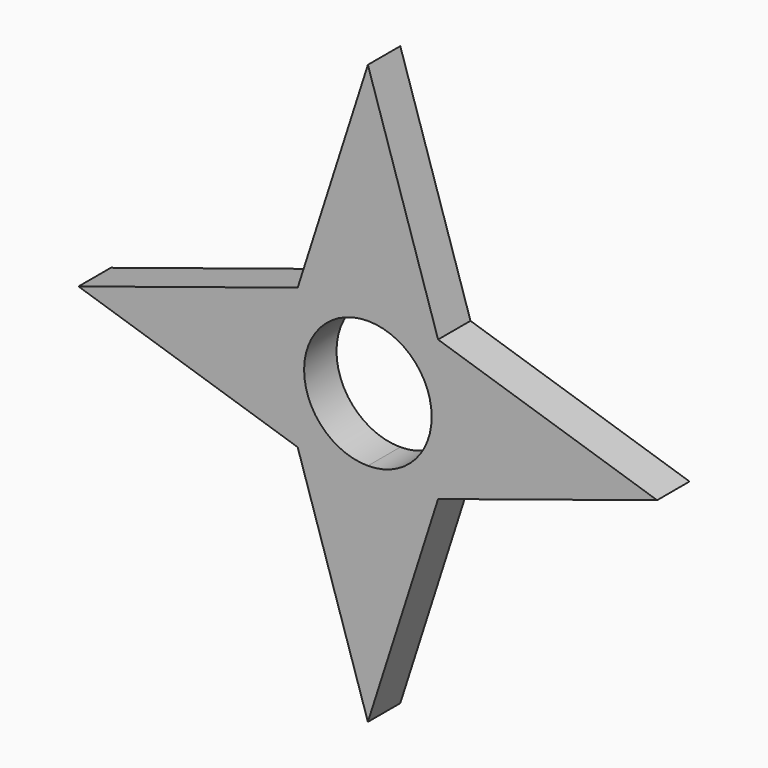
from build123d import *

# Parameters (mm, degrees)
F1_DEPTH = 7


with BuildPart() as f1:
    # F0 (on Front) → F1 (new body)
    with BuildSketch(Plane.XZ):
        with BuildLine():
            Line((13.0394884775, 9.315168557), (16.025, 0))
            ThreePointArc((16.025, 0), (15.2603805302, 4.8909519599), (13.0394884775, 9.315168557))
        make_face()
        with BuildLine():
            ThreePointArc((13.0394884775, 9.315168557), (15.2603805302, 4.8909519599), (16.025, 0))
            ThreePointArc((16.025, 0), (15.2603805302, -4.8909519599), (13.0394884775, -9.315168557))
            Line((13.0394884775, -9.315168557), (12.1355547141, -12.1355547141))
            Line((12.1355547141, -12.1355547141), (50, 0))
            Line((50, 0), (12.1355547141, 12.1355547141))
            Line((12.1355547141, 12.1355547141), (13.0394884775, 9.315168557))
        make_face()
        with BuildLine():
            Line((11.025, 0), (16.025, 0))
            Line((16.025, 0), (13.0394884775, 9.315168557))
            ThreePointArc((13.0394884775, 9.315168557), (11.3313861685, 11.3313861685), (9.315168557, 13.0394884775))
            Line((9.315168557, 13.0394884775), (0, 16.025))
            Line((0, 16.025), (0, 11.025))
            ThreePointArc((0, 11.025), (7.7958522626, 7.7958522626), (11.025, 0))
        make_face()
        with BuildLine():
            ThreePointArc((13.0394884775, -9.315168557), (15.2603805302, -4.8909519599), (16.025, 0))
            Line((16.025, 0), (13.0394884775, -9.315168557))
        make_face()
        with BuildLine():
            Line((13.0394884775, -9.315168557), (16.025, 0))
            Line((16.025, 0), (11.025, 0))
            ThreePointArc((11.025, 0), (7.7958522626, -7.7958522626), (0, -11.025))
            Line((0, -11.025), (0, -16.025))
            Line((0, -16.025), (9.315168557, -13.0394884775))
            ThreePointArc((9.315168557, -13.0394884775), (11.3313861685, -11.3313861685), (13.0394884775, -9.315168557))
        make_face()
        with BuildLine():
            ThreePointArc((9.315168557, 13.0394884775), (11.3313861685, 11.3313861685), (13.0394884775, 9.315168557))
            Line((13.0394884775, 9.315168557), (12.1355547141, 12.1355547141))
            Line((12.1355547141, 12.1355547141), (9.315168557, 13.0394884775))
        make_face()
        with BuildLine():
            Line((12.1355547141, -12.1355547141), (13.0394884775, -9.315168557))
            ThreePointArc((13.0394884775, -9.315168557), (11.3313861685, -11.3313861685), (9.315168557, -13.0394884775))
            Line((9.315168557, -13.0394884775), (12.1355547141, -12.1355547141))
        make_face()
        with BuildLine():
            Line((0, 16.025), (9.315168557, 13.0394884775))
            ThreePointArc((9.315168557, 13.0394884775), (4.8909519599, 15.2603805302), (0, 16.025))
        make_face()
        with BuildLine():
            ThreePointArc((0, 16.025), (4.8909519599, 15.2603805302), (9.315168557, 13.0394884775))
            Line((9.315168557, 13.0394884775), (12.1355547141, 12.1355547141))
            Line((12.1355547141, 12.1355547141), (0, 50))
            Line((0, 50), (-12.1347763783, 12.1379832191))
            Line((-12.1347763783, 12.1379832191), (-9.3109210563, 13.0425217686))
            ThreePointArc((-9.3109210563, 13.0425217686), (-4.8884667156, 15.2611768278), (0, 16.025))
        make_face()
        with BuildLine():
            Line((12.1355547141, -12.1355547141), (9.315168557, -13.0394884775))
            ThreePointArc((9.315168557, -13.0394884775), (4.8909519599, -15.2603805302), (0, -16.025))
            ThreePointArc((0, -16.025), (-4.8884667156, -15.2611768278), (-9.3109210563, -13.0425217686))
            Line((-9.3109210563, -13.0425217686), (-12.1347763783, -12.1379832191))
            Line((-12.1347763783, -12.1379832191), (0, -50))
            Line((0, -50), (12.1355547141, -12.1355547141))
        make_face()
        with BuildLine():
            ThreePointArc((0, -16.025), (4.8909519599, -15.2603805302), (9.315168557, -13.0394884775))
            Line((9.315168557, -13.0394884775), (0, -16.025))
        make_face()
        with BuildLine():
            ThreePointArc((0, -11.025), (-11.025, 0), (0, 11.025))
            Line((0, 11.025), (0, 16.025))
            Line((0, 16.025), (-9.3109210563, 13.0425217686))
            ThreePointArc((-9.3109210563, 13.0425217686), (-11.3295406823, 11.3332313542), (-13.0394884775, 9.315168557))
            Line((-13.0394884775, 9.315168557), (-16.025, 0))
            Line((-16.025, 0), (-13.0394884775, -9.315168557))
            ThreePointArc((-13.0394884775, -9.315168557), (-11.3295406823, -11.3332313542), (-9.3109210563, -13.0425217686))
            Line((-9.3109210563, -13.0425217686), (0, -16.025))
            Line((0, -16.025), (0, -11.025))
        make_face()
        with BuildLine():
            Line((-9.3109210563, 13.0425217686), (0, 16.025))
            ThreePointArc((0, 16.025), (-4.8884667156, 15.2611768278), (-9.3109210563, 13.0425217686))
        make_face()
        with BuildLine():
            ThreePointArc((-9.3109210563, -13.0425217686), (-4.8884667156, -15.2611768278), (0, -16.025))
            Line((0, -16.025), (-9.3109210563, -13.0425217686))
        make_face()
        with BuildLine():
            ThreePointArc((-13.0394884775, 9.315168557), (-11.3295406823, 11.3332313542), (-9.3109210563, 13.0425217686))
            Line((-9.3109210563, 13.0425217686), (-12.1347763783, 12.1379832191))
            Line((-12.1347763783, 12.1379832191), (-13.0394884775, 9.315168557))
        make_face()
        with BuildLine():
            Line((-13.0394884775, 9.315168557), (-12.1347763783, 12.1379832191))
            Line((-12.1347763783, 12.1379832191), (-50.0280298293, 0))
            Line((-50.0280298293, 0), (-12.1347763783, -12.1379832191))
            Line((-12.1347763783, -12.1379832191), (-13.0394884775, -9.315168557))
            ThreePointArc((-13.0394884775, -9.315168557), (-15.2603805302, -4.8909519599), (-16.025, 0))
            ThreePointArc((-16.025, 0), (-15.2603805302, 4.8909519599), (-13.0394884775, 9.315168557))
        make_face()
        with BuildLine():
            Line((-12.1347763783, -12.1379832191), (-9.3109210563, -13.0425217686))
            ThreePointArc((-9.3109210563, -13.0425217686), (-11.3295406823, -11.3332313542), (-13.0394884775, -9.315168557))
            Line((-13.0394884775, -9.315168557), (-12.1347763783, -12.1379832191))
        make_face()
        with BuildLine():
            Line((-16.025, 0), (-13.0394884775, 9.315168557))
            ThreePointArc((-13.0394884775, 9.315168557), (-15.2603805302, 4.8909519599), (-16.025, 0))
        make_face()
        with BuildLine():
            ThreePointArc((-16.025, 0), (-15.2603805302, -4.8909519599), (-13.0394884775, -9.315168557))
            Line((-13.0394884775, -9.315168557), (-16.025, 0))
        make_face()
    extrude(amount=F1_DEPTH)


solid = f1.part
